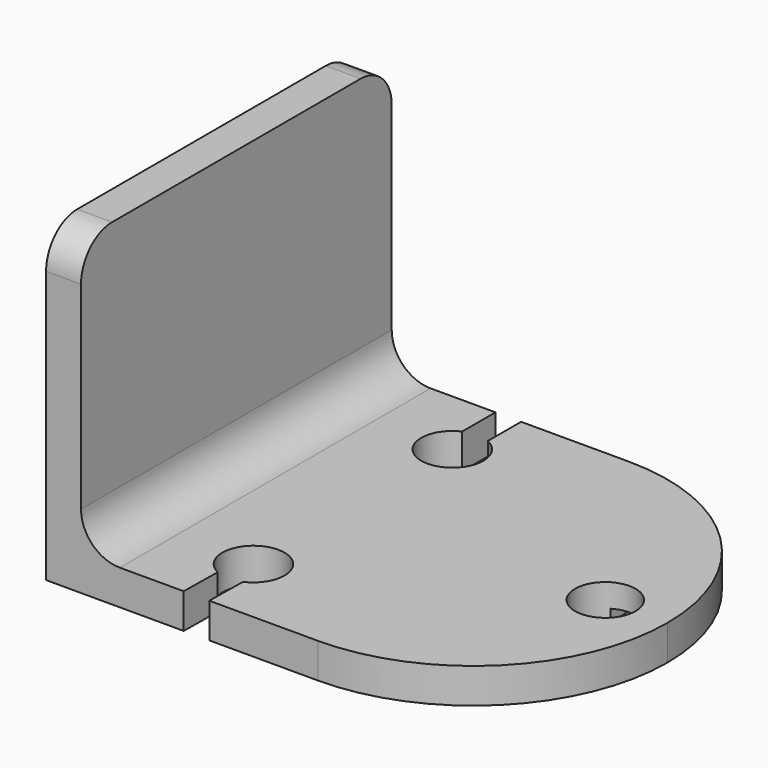
from build123d import *

# Parameters (mm, degrees)
F1_DEPTH  = 50
F2_R      = 25
F3_R      = 24.99999
F4_R      = 3.9
F5_DEPTH  = 12.5
F7_R      = 0.5
F8_DEPTH  = 2.4
F6_R      = 0.5
F9_DEPTH  = 2.4
F11_DEPTH = 1.5
F12_R     = 5
F13_R     = 5
F15_DEPTH = 2.1
F17_DEPTH = 25
F18_DEPTH = 25


# Not quite as in the source:
# - a fillet or chamfer is up to 0.001 mm smaller than in the source, because OpenCascade refuses the exact size
# - ends of sketch curves that miss each other by under 0.0002 mm in the source are joined


with BuildPart() as f1:
    # F0 (on Front) → F1 (new body)
    with BuildSketch(Plane.XZ):
        with BuildLine():
            Line((-24.9614193552, 0), (35.0385806448, 0))
            Line((35.0385806448, 0), (35.0385806448, 4.5))
            Line((35.0385806448, 4.5), (-15.4614193552, 4.5))
            ThreePointArc((-15.4614193552, 4.5), (-18.9969532612, 5.9644660941), (-20.4614193552, 9.5))
            Line((-20.4614193552, 9.5), (-20.4614193552, 40))
            Line((-20.4614193552, 40), (-24.9614193552, 40))
            Line((-24.9614193552, 40), (-24.9614193552, 0))
        make_face()
    extrude(amount=F1_DEPTH)

    # F2
    f2_edges = [f1.edges().sort_by_distance(p)[0] for p in [
        (35.038581, 0, 2.25),
    ]]
    fillet(f2_edges, radius=F2_R)

    # F3 (radius 25 in the source; OpenCascade refuses exactly that, so slightly less here)
    f3_edges = [f1.edges().sort_by_distance(p)[0] for p in [
        (35.038581, -50, 2.25),
    ]]
    fillet(f3_edges, radius=F3_R)

    # F4 (on face) → F5 (cut, symmetric)
    with BuildSketch(Plane.XY.offset(4.5)):
        with Locations((27.0385806448, -25)):
            Circle(F4_R)
    extrude(amount=F5_DEPTH, both=True, mode=Mode.SUBTRACT)

    # F7 (on Top) → F8 (cut, symmetric)
    with BuildSketch(Plane.XY):
        with Locations((27.0385806448, -19)):
            Circle(F7_R)
    extrude(amount=F8_DEPTH, both=True, mode=Mode.SUBTRACT)

    # F6 (on Top) → F9 (cut, symmetric)
    with BuildSketch(Plane.XY):
        with Locations((27.0385806448, -31)):
            Circle(F6_R)
    extrude(amount=F9_DEPTH, both=True, mode=Mode.SUBTRACT)

    # F10 (on Top) → F11 (cut)
    with BuildSketch(Plane.XY):
        with BuildLine():
            Line((25.0421970529, -19.1326886576), (25.0421970529, -30.8567436225))
            ThreePointArc((25.0421970529, -30.8567436225), (27.0370224854, -33.0005194676), (29.031847918, -30.8567436225))
            Line((29.031847918, -30.8567436225), (29.0331744321, -30.8567436225))
            Line((29.0331744321, -30.8567436225), (29.0331744321, -19.1326886576))
            ThreePointArc((29.0331744321, -19.1326886576), (27.0376323306, -16.9991781279), (25.0421970529, -19.1326886576))
        make_face()
    extrude(amount=F11_DEPTH, mode=Mode.SUBTRACT)

    # F12
    f12_edges = [f1.edges().sort_by_distance(p)[0] for p in [
        (-22.711419, -50, 40),
    ]]
    fillet(f12_edges, radius=F12_R)

    # F13
    f13_edges = [f1.edges().sort_by_distance(p)[0] for p in [
        (-22.711419, 0, 40),
    ]]
    fillet(f13_edges, radius=F13_R)

    # F14 (on face) → F15 (cut)
    with BuildSketch(Plane(origin=(-24.9614193552, 0, 0), x_dir=(0, -1, 0), z_dir=(-1, 0, 0))):
        with BuildLine():
            Line((46.8955885446, 23.8107649305), (42.5171071131, 36.1752150642))
            ThreePointArc((42.5171071131, 36.1752150642), (41.1165449237, 37.7616933331), (39.0073708388, 37.93452974))
            Line((39.0073708388, 37.93452974), (33.9392572641, 36.3604687154))
            ThreePointArc((33.9392572641, 36.3604687154), (32.1739564338, 34.3397574907), (32.4926399743, 31.675549977))
            add(Edge.make_bspline(
                [(32.4926399743, 31.675549977), (33.3670492771, 30.3381403961), (35.0987739091, 27.6894664778), (35.7199990478, 23.1066149427), (35.2211127015, 18.2107984297), (33.4472667585, 15.4309330693), (32.5552672148, 14.0330446884)],
                knots=[0, 0, 0, 0, 0.2493081883, 0.4937426091, 0.7454224458, 1, 1, 1, 1], degree=3))
            ThreePointArc((32.5552672148, 14.0330446884), (32.5347631708, 11.4606329376), (34.2782102525, 9.5690423623))
            Line((34.2782102525, 9.5690423623), (39.1331128776, 7.7970703132))
            ThreePointArc((39.1331128776, 7.7970703132), (41.2400733133, 8.0993579825), (42.6161779425, 9.723241033))
            Line((42.6161779425, 9.723241033), (46.8955885446, 21.8079237751))
            ThreePointArc((46.8955885446, 21.8079237751), (47.0676640713, 22.8093443528), (46.8955885446, 23.8107649305))
        make_face()
        with BuildLine():
            ThreePointArc((3.1705893979, 23.8107653384), (2.9985138712, 22.8093447607), (3.1705893979, 21.807924183))
            Line((3.1705893979, 21.807924183), (7.45, 9.723241441))
            ThreePointArc((7.45, 9.723241441), (8.8261046292, 8.0993583904), (10.9330650649, 7.7970707212))
            Line((10.9330650649, 7.7970707212), (15.78796769, 9.5690427702))
            ThreePointArc((15.78796769, 9.5690427702), (17.5314147718, 11.4606333455), (17.5109107277, 14.0330450963))
            add(Edge.make_bspline(
                [(17.5735379682, 31.6755503849), (16.6991286655, 30.3381408041), (14.9674040335, 27.6894668857), (14.3461788947, 23.1066153507), (14.8450652411, 18.2107988376), (16.618911184, 15.4309334772), (17.5109107277, 14.0330450963)],
                knots=[0, 0, 0, 0, 0.2493081883, 0.4937426091, 0.7454224458, 1, 1, 1, 1], degree=3))
            ThreePointArc((17.5735379682, 31.6755503849), (17.8922215087, 34.3397578986), (16.1269206784, 36.3604691233))
            Line((16.1269206784, 36.3604691233), (11.0588071037, 37.9345301479))
            ThreePointArc((11.0588071037, 37.9345301479), (8.9496330188, 37.7616937411), (7.5490708294, 36.1752154721))
            Line((7.5490708294, 36.1752154721), (3.1705893979, 23.8107653384))
        make_face()
    extrude(amount=-F15_DEPTH, mode=Mode.SUBTRACT)

    # F16 (on Top) → F17 (cut)
    with BuildSketch(Plane.XY):
        with BuildLine():
            Line((-7.103768643, 0), (-7.1083206196, -5.3547680149))
            ThreePointArc((-7.1083206196, -5.3547680149), (-5.4648196706, -12.9999985547), (-3.8083230043, -5.357573274))
            Line((-3.8083230043, -5.357573274), (-3.803768643, 0))
            Line((-3.803768643, 0), (-7.103768643, 0))
        make_face()
        with BuildLine():
            Line((-3.9466372691, -50.0011853874), (-3.8665251866, -44.6682846933))
            ThreePointArc((-3.8665251866, -44.6682846933), (-5.4013371978, -37.0004512587), (-7.1657806518, -44.6187225054))
            Line((-7.1657806518, -44.6187225054), (-7.2466372691, -50.0011853874))
            Line((-7.2466372691, -50.0011853874), (-3.9466372691, -50.0011853874))
        make_face()
    extrude(amount=F17_DEPTH, mode=Mode.SUBTRACT)

    # F16 (on Top) → F18 (cut)
    with BuildSketch(Plane.XY):
        with BuildLine():
            Line((-7.103768643, 0), (-7.1083206196, -5.3547680149))
            ThreePointArc((-7.1083206196, -5.3547680149), (-5.4648196706, -12.9999985547), (-3.8083230043, -5.357573274))
            Line((-3.8083230043, -5.357573274), (-3.803768643, 0))
            Line((-3.803768643, 0), (-7.103768643, 0))
        make_face()
        with BuildLine():
            Line((-3.9466372691, -50.0011853874), (-3.8665251866, -44.6682846933))
            ThreePointArc((-3.8665251866, -44.6682846933), (-5.4013371978, -37.0004512587), (-7.1657806518, -44.6187225054))
            Line((-7.1657806518, -44.6187225054), (-7.2466372691, -50.0011853874))
            Line((-7.2466372691, -50.0011853874), (-3.9466372691, -50.0011853874))
        make_face()
    extrude(amount=F18_DEPTH, mode=Mode.SUBTRACT)


solid = f1.part
